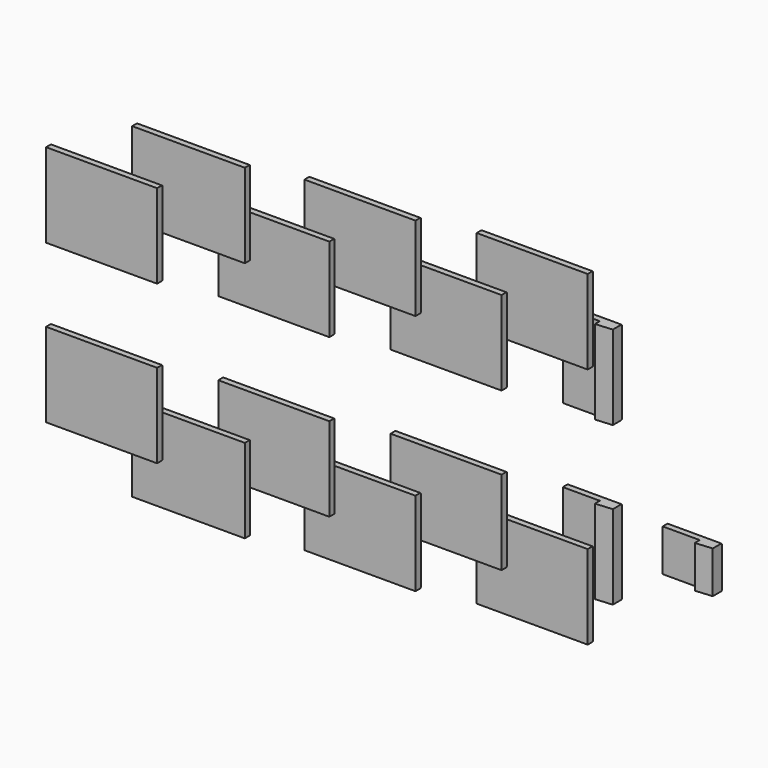
from build123d import *

# Parameters (mm, degrees)
F0_W          = 419.1
F0_H          = 25.4
F1_DEPTH      = 317.5
F2_SIZE       = 2.54
F2_2_SIZE     = 2.54
F2_3_SIZE     = 2.54
F2_4_SIZE     = 2.54
F4_W          = 425.2820260142
F4_H          = 25.4
F5_DEPTH      = 311.15
F5_DEPTH_BACK = 6.35
F4_W_2        = 419.1
F4_H_2        = 25.3773033619
F6_SIZE       = 2.54
F6_2_SIZE     = 2.54
F6_3_SIZE     = 2.54
F8_DEPTH      = 158.75
F9_SIZE       = 2.54


# Not quite as in the source:
# - a feature names something its author has since deleted; it is built from what else it names


with BuildPart() as f1:
    # F0 (on Top) → F1 (new body)
    with BuildSketch(Plane.XY):
        with Locations((209.55, 12.7)):
            Rectangle(F0_W, F0_H)
    extrude(amount=F1_DEPTH)

    # F2
    f2_edges = [f1.edges().sort_by_distance(p)[0] for p in [
        (209.55, 25.4, 317.5),
        (209.55, 25.4, 0),
    ]]
    chamfer(f2_edges, length=F2_SIZE)


with BuildPart() as f1b:
    # F0 (on Top) → F1, piece 2 (new body)
    with BuildSketch(Plane.XY):
        with Locations((819.15, 63.5)):
            Rectangle(F0_W, F0_H)
    extrude(amount=F1_DEPTH)

    # F2#2
    f2_2_edges = [f1b.edges().sort_by_distance(p)[0] for p in [
        (819.15, 76.2, 317.5),
        (819.15, 76.2, 0),
    ]]
    chamfer(f2_2_edges, length=F2_2_SIZE)


with BuildPart() as f1c:
    # F0 (on Top) → F1, piece 3 (new body)
    with BuildSketch(Plane.XY):
        with Locations((1428.75, 114.3)):
            Rectangle(F0_W, F0_H)
    extrude(amount=F1_DEPTH)

    # F2#3
    f2_3_edges = [f1c.edges().sort_by_distance(p)[0] for p in [
        (1428.75, 127, 317.5),
        (1428.75, 127, 0),
    ]]
    chamfer(f2_3_edges, length=F2_3_SIZE)


with BuildPart() as f1d:
    # F0 (on Top) → F1, piece 4 (new body)
    with BuildSketch(Plane.XY):
        Polygon((1968.5, 152.4), (1968.5, 129.1166666667), (2032, 134.4083333333), (2032, 177.8), (1828.8, 177.8), (1828.8, 152.4), align=None)
    extrude(amount=F1_DEPTH)

    # F2#4
    f2_4_edges = [f1d.edges().sort_by_distance(p)[0] for p in [
        (1930.4, 177.8, 317.5),
        (1930.4, 177.8, 0),
    ]]
    chamfer(f2_4_edges, length=F2_4_SIZE)


with BuildPart() as f5:
    # F4 (on offset) → F5 (new body, two sides)
    with BuildSketch(Plane.XY.offset(152.4)) as f5_sk:
        with Locations((517.4410130071, 38.1)):
            Rectangle(F4_W, F4_H)
    extrude(amount=-F5_DEPTH)
    extrude(f5_sk.sketch, amount=F5_DEPTH_BACK)

    # F6
    f6_edges = [f5.edges().sort_by_distance(p)[0] for p in [
        (517.441013, 50.8, 158.75),
        (517.441013, 50.8, -158.75),
    ]]
    chamfer(f6_edges, length=F6_SIZE)


with BuildPart() as f5b:
    # F4 (on offset) → F5, piece 2 (new body, two sides)
    with BuildSketch(Plane.XY.offset(152.4)) as f5_2_sk:
        with Locations((1123.95, 88.9)):
            Rectangle(F4_W_2, F4_H)
    extrude(amount=-F5_DEPTH)
    extrude(f5_2_sk.sketch, amount=F5_DEPTH_BACK)

    # F6#2
    f6_2_edges = [f5b.edges().sort_by_distance(p)[0] for p in [
        (1123.95, 101.6, -158.75),
        (1123.95, 101.6, 158.75),
    ]]
    chamfer(f6_2_edges, length=F6_2_SIZE)


with BuildPart() as f5c:
    # F4 (on offset) → F5, piece 3 (new body, two sides)
    with BuildSketch(Plane.XY.offset(152.4)) as f5_3_sk:
        with Locations((1733.55, 139.8095786572)):
            Rectangle(F4_W_2, F4_H_2)
    extrude(amount=-F5_DEPTH)
    extrude(f5_3_sk.sketch, amount=F5_DEPTH_BACK)

    # F6#3
    f6_3_edges = [f5c.edges().sort_by_distance(p)[0] for p in [
        (1733.55, 152.49823, -158.75),
        (1733.55, 152.49823, 158.75),
    ]]
    chamfer(f6_3_edges, length=F6_3_SIZE)


with BuildPart() as f8:
    # F7 (on face) → F8 (new body)
    with BuildSketch(Plane.XY.offset(317.5)):
        Polygon((2418.7764174887, 165.8460989008), (2215.5764174887, 165.8460989008), (2215.5764174887, 140.4460989008), (2355.2764174887, 140.4460989008), (2355.2764174887, 117.1542989008), (2418.7764174887, 122.4628989008), align=None)
    extrude(amount=-F8_DEPTH)

    # F9
    f9_edges = [f8.edges().sort_by_distance(p)[0] for p in [
        (2317.176417, 165.846099, 317.5),
        (2317.176417, 165.846099, 158.75),
    ]]
    chamfer(f9_edges, length=F9_SIZE)


with BuildPart() as f11_1:
    # F11: instance of F5c
    add(f5c.part.mirror(Plane.XY.offset(457.2)))


with BuildPart() as f11_2:
    # F11: instance of F5b
    add(f5b.part.mirror(Plane.XY.offset(457.2)))


with BuildPart() as f11_3:
    # F11: instance of F5
    add(f5.part.mirror(Plane.XY.offset(457.2)))


with BuildPart() as f11_4:
    # F11: instance of F1d
    add(f1d.part.mirror(Plane.XY.offset(457.2)))


with BuildPart() as f11_5:
    # F11: instance of F1c
    add(f1c.part.mirror(Plane.XY.offset(457.2)))


with BuildPart() as f11_6:
    # F11: instance of F1b
    add(f1b.part.mirror(Plane.XY.offset(457.2)))


with BuildPart() as f11_7:
    # F11: instance of F1
    add(f1.part.mirror(Plane.XY.offset(457.2)))


solid = Compound([f1.part, f1b.part, f1c.part, f1d.part, f5.part, f5b.part, f5c.part, f8.part, f11_1.part, f11_2.part, f11_3.part, f11_4.part, f11_5.part, f11_6.part, f11_7.part])
